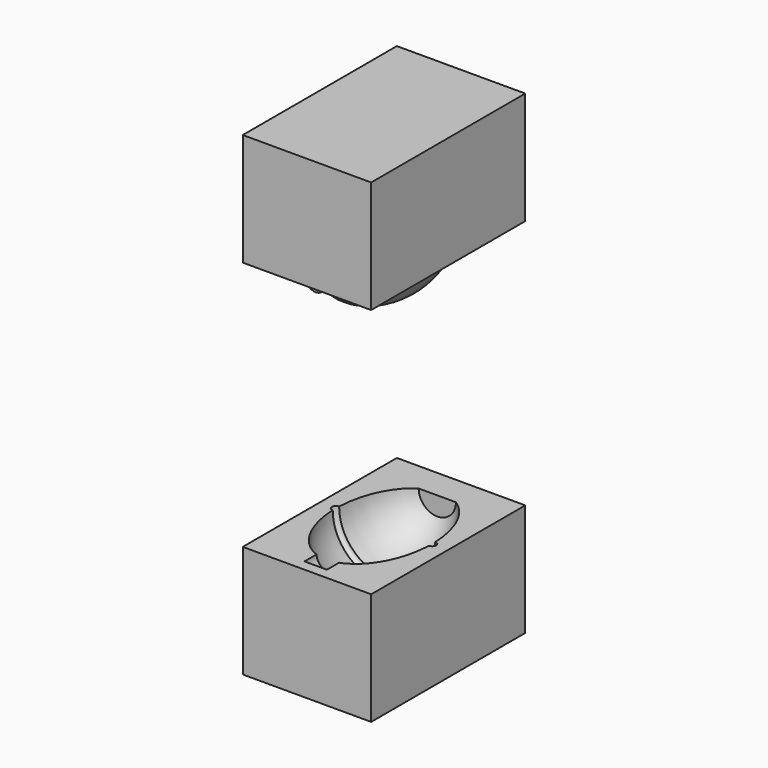
from build123d import *

# Parameters (mm, degrees)
F0_W     = 80
F0_H     = 120
F2_DEPTH = 70
F8_ANGLE = 180


# Not quite as in the source:
# - a feature names something its author has since deleted; it is built from what else it names


with BuildPart() as f2:
    # F0 (on Top) → F2 (new body)
    with BuildSketch(Plane.XY):
        Rectangle(F0_W, F0_H)
        with BuildLine():
            add(Edge.make_bspline(
                [(11.5998084275, -41.5), (96.1455069835, 11.6712359011), (7, 43.7578564374)],
                knots=[0.3970074492, 0.3970074492, 0.3970074492, 2.9060884169, 2.9060884169, 2.9060884169], degree=2, weights=[1, 0.3110102775, 1]))
            Line((11.5998084275, -41.5), (20, -41.5))
            Line((20, -41.5), (20, -48.5))
            Line((20, -48.5), (-20, -48.5))
            Line((-20, -48.5), (-20, -41.5))
            Line((-20, -41.5), (-11.5998084275, -41.5))
            add(Edge.make_bspline(
                [(-29.9536838409, -2.4995709259), (-28.911018824, -30.6128884444), (-11.5998084275, -41.5)],
                knots=[4.7679636039, 4.7679636039, 4.7679636039, 5.886177858, 5.886177858, 5.886177858], degree=2, weights=[1, 0.847729055, 1]))
            ThreePointArc((-29.9536838409, -2.4995709259), (-32.5, 0), (-29.9536838409, 2.4995709259))
            add(Edge.make_bspline(
                [(-7, 43.7578564374), (-28.7133563077, 35.9424516235), (-29.9536838409, 2.4995709259)],
                knots=[3.3770968903, 3.3770968903, 3.3770968903, 4.6568143568, 4.6568143568, 4.6568143568], degree=2, weights=[1, 0.8021801137, 1]))
            Line((-7, 43.7578564374), (-7, 53.1927423179))
            Line((-7, 53.1927423179), (0, 53.1927423179))
            Line((0, 53.1927423179), (7, 53.1927423179))
            Line((7, 53.1927423179), (7, 43.7578564374))
        make_face(mode=Mode.SUBTRACT)
        with BuildLine():
            Line((0, -41.5), (11.5998084275, -41.5))
            add(Edge.make_bspline(
                [(11.5998084275, -41.5), (96.1455069835, 11.6712359011), (7, 43.7578564374)],
                knots=[0.3970074492, 0.3970074492, 0.3970074492, 2.9060884169, 2.9060884169, 2.9060884169], degree=2, weights=[1, 0.3110102775, 1]))
            Line((7, 43.7578564374), (7, 36.8072576821))
            Line((7, 36.8072576821), (0, 36.8072576821))
            Line((0, 36.8072576821), (0, -41.5))
        make_face()
        with BuildLine():
            add(Edge.make_bspline(
                [(-29.9536838409, -2.4995709259), (-28.911018824, -30.6128884444), (-11.5998084275, -41.5)],
                knots=[4.7679636039, 4.7679636039, 4.7679636039, 5.886177858, 5.886177858, 5.886177858], degree=2, weights=[1, 0.847729055, 1]))
            Line((-11.5998084275, -41.5), (0, -41.5))
            Line((0, -41.5), (0, 36.8072576821))
            Line((0, 36.8072576821), (-7, 36.8072576821))
            Line((-7, 36.8072576821), (-7, 43.7578564374))
            add(Edge.make_bspline(
                [(-7, 43.7578564374), (-28.7133563077, 35.9424516235), (-29.9536838409, 2.4995709259)],
                knots=[3.3770968903, 3.3770968903, 3.3770968903, 4.6568143568, 4.6568143568, 4.6568143568], degree=2, weights=[1, 0.8021801137, 1]))
            ThreePointArc((-29.9536838409, 2.4995709259), (-28.2159329612, 1.7513151633), (-27.5, 0))
            ThreePointArc((-27.5, 0), (-28.2159329612, -1.7513151633), (-29.9536838409, -2.4995709259))
        make_face()
        with BuildLine():
            Line((7, 36.8072576821), (7, 43.7578564374))
            add(Edge.make_bspline(
                [(7, 43.7578564374), (3.5489816073, 45), (0, 45)],
                knots=[2.9060884169, 2.9060884169, 2.9060884169, 3.1415926536, 3.1415926536, 3.1415926536], degree=2, weights=[1, 0.9930752262, 1]))
            Line((0, 45), (0, 36.8072576821))
            Line((0, 36.8072576821), (7, 36.8072576821))
        make_face()
        with BuildLine():
            Line((-7, 36.8072576821), (0, 36.8072576821))
            Line((0, 36.8072576821), (0, 45))
            add(Edge.make_bspline(
                [(0, 45), (-3.5489816073, 45), (-7, 43.7578564374)],
                knots=[3.1415926536, 3.1415926536, 3.1415926536, 3.3770968903, 3.3770968903, 3.3770968903], degree=2, weights=[1, 0.9930752262, 1]))
            Line((-7, 43.7578564374), (-7, 36.8072576821))
        make_face()
        with BuildLine():
            add(Edge.make_bspline(
                [(7, 43.7578564374), (3.5489816073, 45), (0, 45)],
                knots=[2.9060884169, 2.9060884169, 2.9060884169, 3.1415926536, 3.1415926536, 3.1415926536], degree=2, weights=[1, 0.9930752262, 1]))
            Line((7, 43.7578564374), (7, 53.1927423179))
            Line((7, 53.1927423179), (0, 53.1927423179))
            Line((0, 53.1927423179), (0, 45))
        make_face()
        with BuildLine():
            add(Edge.make_bspline(
                [(0, 45), (-3.5489816073, 45), (-7, 43.7578564374)],
                knots=[3.1415926536, 3.1415926536, 3.1415926536, 3.3770968903, 3.3770968903, 3.3770968903], degree=2, weights=[1, 0.9930752262, 1]))
            Line((0, 45), (0, 53.1927423179))
            Line((0, 53.1927423179), (-7, 53.1927423179))
            Line((-7, 53.1927423179), (-7, 43.7578564374))
        make_face()
        with BuildLine():
            ThreePointArc((-29.9536838409, 2.4995709259), (-32.5, 0), (-29.9536838409, -2.4995709259))
            add(Edge.make_bspline(
                [(-29.9536838409, 2.4995709259), (-30.0463877759, 0), (-29.9536838409, -2.4995709259)],
                knots=[4.6568143568, 4.6568143568, 4.6568143568, 4.7679636039, 4.7679636039, 4.7679636039], degree=2, weights=[1, 0.998456128, 1]))
        make_face()
        with BuildLine():
            add(Edge.make_bspline(
                [(-29.9536838409, 2.4995709259), (-30.0463877759, 0), (-29.9536838409, -2.4995709259)],
                knots=[4.6568143568, 4.6568143568, 4.6568143568, 4.7679636039, 4.7679636039, 4.7679636039], degree=2, weights=[1, 0.998456128, 1]))
            ThreePointArc((-29.9536838409, -2.4995709259), (-28.2159329612, -1.7513151633), (-27.5, 0))
            ThreePointArc((-27.5, 0), (-28.2159329612, 1.7513151633), (-29.9536838409, 2.4995709259))
        make_face()
        with BuildLine():
            Line((0, -41.5), (0, -45))
            add(Edge.make_bspline(
                [(0, -45), (6.0345824189, -45), (11.5998084275, -41.5)],
                knots=[0, 0, 0, 0.3970074492, 0.3970074492, 0.3970074492], degree=2, weights=[1, 0.9803627447, 1]))
            Line((11.5998084275, -41.5), (0, -41.5))
        make_face()
        with BuildLine():
            add(Edge.make_bspline(
                [(0, -45), (6.0345824189, -45), (11.5998084275, -41.5)],
                knots=[0, 0, 0, 0.3970074492, 0.3970074492, 0.3970074492], degree=2, weights=[1, 0.9803627447, 1]))
            add(Edge.make_bspline(
                [(-11.5998084275, -41.5), (-6.0345824189, -45), (0, -45)],
                knots=[5.886177858, 5.886177858, 5.886177858, 6.2831853072, 6.2831853072, 6.2831853072], degree=2, weights=[1, 0.9803627447, 1]))
            Line((-11.5998084275, -41.5), (-20, -41.5))
            Line((-20, -41.5), (-20, -48.5))
            Line((-20, -48.5), (20, -48.5))
            Line((20, -48.5), (20, -41.5))
            Line((20, -41.5), (11.5998084275, -41.5))
        make_face()
        with BuildLine():
            add(Edge.make_bspline(
                [(-11.5998084275, -41.5), (-6.0345824189, -45), (0, -45)],
                knots=[5.886177858, 5.886177858, 5.886177858, 6.2831853072, 6.2831853072, 6.2831853072], degree=2, weights=[1, 0.9803627447, 1]))
            Line((0, -45), (0, -41.5))
            Line((0, -41.5), (-11.5998084275, -41.5))
        make_face()
    extrude(amount=F2_DEPTH)


with BuildPart() as f3_1:
    # F3: copy of F2
    add(f2.part.moved(Location((0, 0, 155.9))))

    # F5 (on face) → F6 (revolve)
    with BuildSketch(Plane(origin=(0, 0, 155.9), x_dir=(1, 0, 0), z_dir=(0, 0, -1))):
        with BuildLine():
            add(Edge.make_bspline(
                [(-5.9999991059, 43.0479642897), (-96.1289526789, 14.1296936695), (-11.3346382454, -40.5)],
                knots=[3.3499944602, 3.3499944602, 3.3499944602, 5.8816308452, 5.8816308452, 5.8816308452], degree=2, weights=[1, 0.3002723186, 1]))
            Line((-11.3346382454, -40.5), (8.941e-07, -40.5))
            Line((8.941e-07, -40.5), (8.941e-07, 34.80726))
            Line((8.941e-07, 34.80726), (-5.9999991059, 34.80726))
            Line((-5.9999991059, 34.80726), (-5.9999991059, 43.0479642897))
        make_face()
        with BuildLine():
            add(Edge.make_bspline(
                [(8.941e-07, 44), (-3.0328098345, 44), (-5.9999991059, 43.0479642897)],
                knots=[3.1415926536, 3.1415926536, 3.1415926536, 3.3499944602, 3.3499944602, 3.3499944602], degree=2, weights=[1, 0.9945759963, 1]))
            Line((-5.9999991059, 43.0479642897), (-5.9999991059, 34.80726))
            Line((-5.9999991059, 34.80726), (8.941e-07, 34.80726))
            Line((8.941e-07, 34.80726), (8.941e-07, 44))
        make_face()
        with BuildLine():
            Line((-5.9999991059, 53.19274), (-5.9999991059, 43.0479642897))
            add(Edge.make_bspline(
                [(8.941e-07, 44), (-3.0328098345, 44), (-5.9999991059, 43.0479642897)],
                knots=[3.1415926536, 3.1415926536, 3.1415926536, 3.3499944602, 3.3499944602, 3.3499944602], degree=2, weights=[1, 0.9945759963, 1]))
            Line((8.941e-07, 44), (8.941e-07, 53.19274))
            Line((8.941e-07, 53.19274), (-5.9999991059, 53.19274))
        make_face()
    revolve(axis=Axis((8.941e-07, -4.59637, 155.9), (0, -1, 0)))


with BuildPart() as f2_1:
    add(f2.part)

    # F0 (on Top) → F4 (revolve, cut)
    with BuildSketch(Plane.XY):
        with BuildLine():
            add(Edge.make_bspline(
                [(-29.9536838409, -2.4995709259), (-28.911018824, -30.6128884444), (-11.5998084275, -41.5)],
                knots=[4.7679636039, 4.7679636039, 4.7679636039, 5.886177858, 5.886177858, 5.886177858], degree=2, weights=[1, 0.847729055, 1]))
            Line((-11.5998084275, -41.5), (0, -41.5))
            Line((0, -41.5), (0, 36.8072576821))
            Line((0, 36.8072576821), (-7, 36.8072576821))
            Line((-7, 36.8072576821), (-7, 43.7578564374))
            add(Edge.make_bspline(
                [(-7, 43.7578564374), (-28.7133563077, 35.9424516235), (-29.9536838409, 2.4995709259)],
                knots=[3.3770968903, 3.3770968903, 3.3770968903, 4.6568143568, 4.6568143568, 4.6568143568], degree=2, weights=[1, 0.8021801137, 1]))
            ThreePointArc((-29.9536838409, 2.4995709259), (-28.2159329612, 1.7513151633), (-27.5, 0))
            ThreePointArc((-27.5, 0), (-28.2159329612, -1.7513151633), (-29.9536838409, -2.4995709259))
        make_face()
        with BuildLine():
            add(Edge.make_bspline(
                [(-29.9536838409, 2.4995709259), (-30.0463877759, 0), (-29.9536838409, -2.4995709259)],
                knots=[4.6568143568, 4.6568143568, 4.6568143568, 4.7679636039, 4.7679636039, 4.7679636039], degree=2, weights=[1, 0.998456128, 1]))
            ThreePointArc((-29.9536838409, -2.4995709259), (-28.2159329612, -1.7513151633), (-27.5, 0))
            ThreePointArc((-27.5, 0), (-28.2159329612, 1.7513151633), (-29.9536838409, 2.4995709259))
        make_face()
        with BuildLine():
            ThreePointArc((-29.9536838409, 2.4995709259), (-32.5, 0), (-29.9536838409, -2.4995709259))
            add(Edge.make_bspline(
                [(-29.9536838409, 2.4995709259), (-30.0463877759, 0), (-29.9536838409, -2.4995709259)],
                knots=[4.6568143568, 4.6568143568, 4.6568143568, 4.7679636039, 4.7679636039, 4.7679636039], degree=2, weights=[1, 0.998456128, 1]))
        make_face()
        with BuildLine():
            Line((-7, 36.8072576821), (0, 36.8072576821))
            Line((0, 36.8072576821), (0, 45))
            add(Edge.make_bspline(
                [(0, 45), (-3.5489816073, 45), (-7, 43.7578564374)],
                knots=[3.1415926536, 3.1415926536, 3.1415926536, 3.3770968903, 3.3770968903, 3.3770968903], degree=2, weights=[1, 0.9930752262, 1]))
            Line((-7, 43.7578564374), (-7, 36.8072576821))
        make_face()
        with BuildLine():
            add(Edge.make_bspline(
                [(0, 45), (-3.5489816073, 45), (-7, 43.7578564374)],
                knots=[3.1415926536, 3.1415926536, 3.1415926536, 3.3770968903, 3.3770968903, 3.3770968903], degree=2, weights=[1, 0.9930752262, 1]))
            Line((0, 45), (0, 53.1927423179))
            Line((0, 53.1927423179), (-7, 53.1927423179))
            Line((-7, 53.1927423179), (-7, 43.7578564374))
        make_face()
    revolve(axis=Axis((0, 4.096371159, 0), (0, 1, 0)), mode=Mode.SUBTRACT)


with BuildPart() as f2_2:
    # F8: moved
    add(f2_1.part.rotate(Axis((0.2401061356, 0, 0), (1, 0, 0)), F8_ANGLE))


solid = Compound([f3_1.part, f2_2.part])
